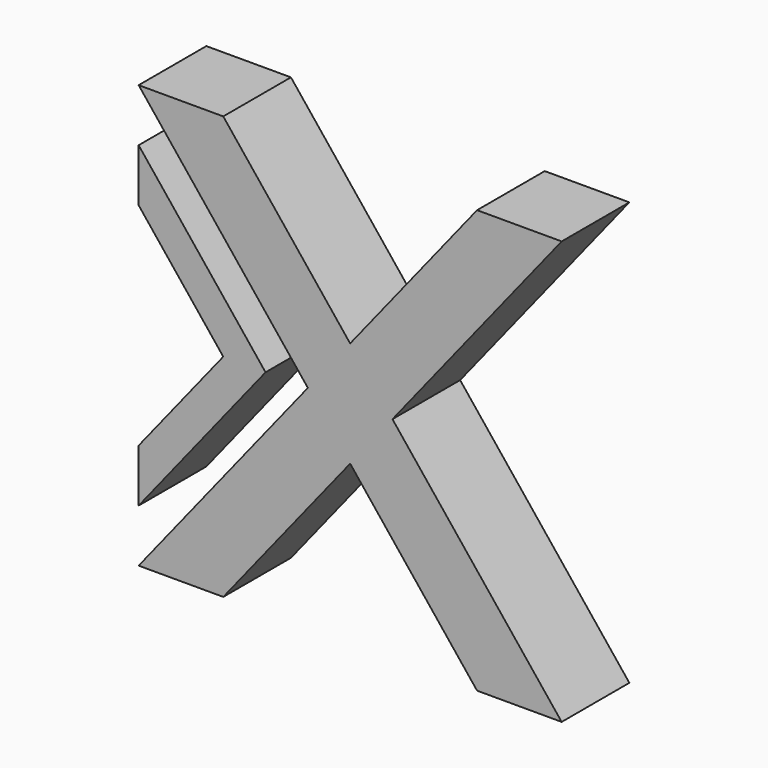
from build123d import *

# Parameters (mm, degrees)
F3_DEPTH = 121.92


# Not quite as in the source:
# - a variable given as a bare number and used for a length is read in inches; the dataset says mm whatever the document's units were


with BuildPart() as f3:
    # F2 (on Front) → F3 (new body)
    with BuildSketch(Plane.XZ):
        Polygon((60.96, 0), (304.8, 304.8), (182.88, 304.8), (0, 76.2), (-182.88, 304.8), (-304.8, 304.8), (-60.96, 0), (-304.8, -304.8), (-182.88, -304.8), (0, -76.2), (182.88, -304.8), (304.8, -304.8), align=None)
    extrude(amount=F3_DEPTH)


with BuildPart() as f3b:
    # F2 (on Front) → F3, piece 2 (new body)
    with BuildSketch(Plane.XZ):
        Polygon((-121.92, 0), (-304.8, 228.6), (-304.8, 152.4), (-182.88, 0), (-304.8, -152.4), (-304.8, -228.6), align=None)
    extrude(amount=F3_DEPTH)


solid = Compound([f3.part, f3b.part])
